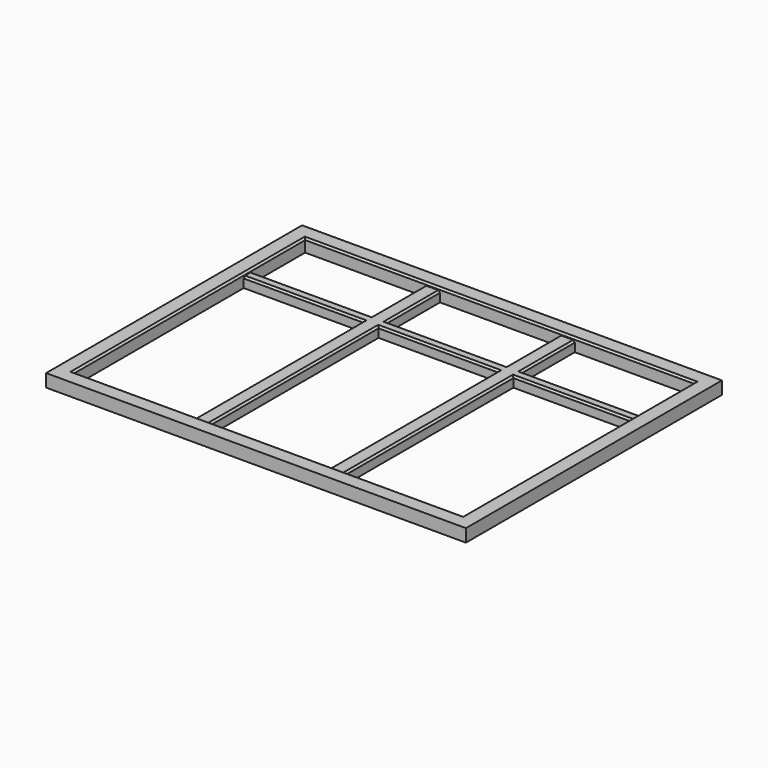
from build123d import *

# Parameters (mm, degrees)
F0_W      = 1640
F0_H      = 1250
F1_DEPTH  = 50
F2_DEPTH  = 40
F3_SIZE   = 7
F3_2_SIZE = 7


# Not quite as in the source:
# - a feature names something its author has since deleted; it is built from what else it names


with BuildPart() as f1:
    # F0 (on Top) → F1 (new body)
    with BuildSketch(Plane.XY):
        with Locations((502.9808287794, 90.2047318473)):
            Rectangle(F0_W, F0_H)
        Polygon((-257.0191712206, 395.2047318473), (-257.0191712206, 655.2047318473), (209.6474954461, 655.2047318473), (269.6474954461, 655.2047318473), (736.3141621128, 655.2047318473), (796.3141621128, 655.2047318473), (1262.9808287794, 655.2047318473), (1262.9808287794, 395.2047318473), (1262.9808287794, 355.2047318473), (1262.9808287794, -474.7952681527), (796.3141621128, -474.7952681527), (736.3141621128, -474.7952681527), (269.6474954461, -474.7952681527), (209.6474954461, -474.7952681527), (-257.0191712206, -474.7952681527), (-257.0191712206, 355.2047318473), align=None, mode=Mode.SUBTRACT)
    extrude(amount=F1_DEPTH)

    # F3
    f3_edges = [f1.edges().sort_by_distance(p)[0] for p in [
        (-257.019171, 90.204732, 50),
        (502.980829, 655.204732, 50),
        (502.980829, -474.795268, 50),
        (1262.980829, 90.204732, 50),
    ]]
    chamfer(f3_edges, length=F3_SIZE)


with BuildPart() as f2:
    # F0 (on Top) → F2 (new body)
    with BuildSketch(Plane.XY):
        Polygon((269.6474954461, 655.2047318473), (209.6474954461, 655.2047318473), (209.6474954461, 395.2047318473), (-257.0191712206, 395.2047318473), (-257.0191712206, 355.2047318473), (209.6474954461, 355.2047318473), (209.6474954461, -474.7952681527), (269.6474954461, -474.7952681527), (269.6474954461, 355.2047318473), (736.3141621128, 355.2047318473), (736.3141621128, -474.7952681527), (796.3141621128, -474.7952681527), (796.3141621128, 355.2047318473), (1262.9808287794, 355.2047318473), (1262.9808287794, 395.2047318473), (796.3141621128, 395.2047318473), (796.3141621128, 655.2047318473), (736.3141621128, 655.2047318473), (736.3141621128, 395.2047318473), (269.6474954461, 395.2047318473), align=None)
    extrude(amount=F2_DEPTH)

    # F3#2
    f3_2_edges = [f2.edges().sort_by_distance(p)[0] for p in [
        (-23.685838, 355.204732, 40),
        (502.980829, 355.204732, 40),
        (269.647495, -59.795268, 40),
        (796.314162, -59.795268, 40),
        (796.314162, 525.204732, 40),
        (269.647495, 525.204732, 40),
        (209.647495, -59.795268, 40),
        (209.647495, 525.204732, 40),
        (-23.685838, 395.204732, 40),
        (502.980829, 395.204732, 40),
        (1029.647495, 395.204732, 40),
        (1029.647495, 355.204732, 40),
        (736.314162, -59.795268, 40),
        (736.314162, 525.204732, 40),
    ]]
    chamfer(f3_2_edges, length=F3_2_SIZE)


solid = Compound([f1.part, f2.part])
